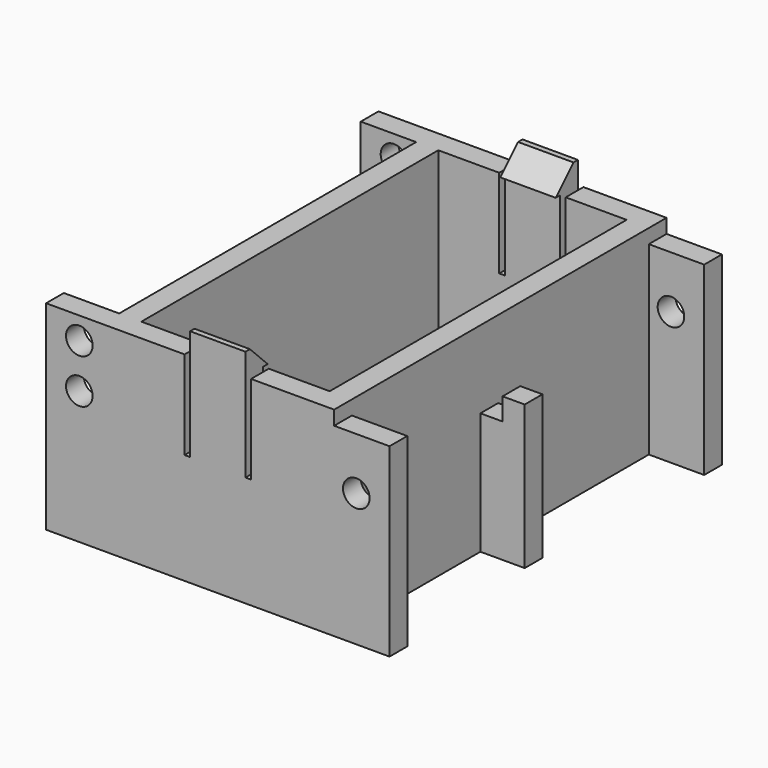
from build123d import *

# Parameters (mm, degrees)
F1_DEPTH  = 2
F2_DEPTH  = 18
F3_DEPTH  = 3
F4_W      = 2
F4_H      = 5
F4_H_2    = 13
F5_DEPTH  = 5
F6_W      = 2
F6_H      = 16.7173967883
F7_DEPTH  = 5
F8_R      = 1.2
F9_DEPTH  = 40
F12_DEPTH = 1
F13_W     = 5
F13_H     = 2
F13_H_2   = 0.5
F14_DEPTH = 2
F15_SIZE  = 1.99999
F13_W_2   = 0.5
F16_DEPTH = 8


# Not quite as in the source:
# - a fillet or chamfer is up to 0.001 mm smaller than in the source, because OpenCascade refuses the exact size


with BuildPart() as f1:
    # F0 (on Top) → F1 (new body)
    with BuildSketch(Plane.XY):
        Polygon((-5.1606558692, 9.7513413054), (-11.6606558692, 9.7513413054), (-11.6606558692, -27.7486586946), (-5.1606558692, -27.7486586946), (2.8393441308, -27.7486586946), (9.3393441308, -27.7486586946), (9.3393441308, 9.7513413054), (2.8393441308, 9.7513413054), align=None)
        Polygon((-9.6606558692, -1.2486586946), (-9.6606558692, 7.7513413054), (7.3393441308, 7.7513413054), (7.3393441308, -1.2486586946), (7.3393441308, -16.7486586946), (7.3393441308, -25.7486586946), (-9.6606558692, -25.7486586946), (-9.6606558692, -16.7486586946), align=None, mode=Mode.SUBTRACT)
        with BuildLine():
            Line((3.3125979801, -16.7486586946), (-5.6339097184, -16.7486586946))
            ThreePointArc((-5.6339097184, -16.7486586946), (-2.8409986659, -25.1856853401), (4.3393441308, -19.9486586946))
            ThreePointArc((4.3393441308, -19.9486586946), (4.0763707763, -18.2683158979), (3.3125979801, -16.7486586946))
        make_face()
        with BuildLine():
            ThreePointArc((4.3393441308, 1.9513413054), (-2.8409986659, 7.1883679509), (-5.6339097184, -1.2486586946))
            Line((-5.6339097184, -1.2486586946), (3.3125979801, -1.2486586946))
            ThreePointArc((3.3125979801, -1.2486586946), (4.0763707763, 0.2709985087), (4.3393441308, 1.9513413054))
        make_face()
        with BuildLine():
            Line((7.3393441308, 7.7513413054), (-9.6606558692, 7.7513413054))
            Line((-9.6606558692, 7.7513413054), (-9.6606558692, -1.2486586946))
            Line((-9.6606558692, -1.2486586946), (-5.6339097184, -1.2486586946))
            ThreePointArc((-5.6339097184, -1.2486586946), (-2.8409986659, 7.1883679509), (4.3393441308, 1.9513413054))
            ThreePointArc((4.3393441308, 1.9513413054), (4.0763707763, 0.2709985087), (3.3125979801, -1.2486586946))
            Line((3.3125979801, -1.2486586946), (7.3393441308, -1.2486586946))
            Line((7.3393441308, -1.2486586946), (7.3393441308, 7.7513413054))
        make_face()
        with BuildLine():
            Line((-5.6339097184, -16.7486586946), (-9.6606558692, -16.7486586946))
            Line((-9.6606558692, -16.7486586946), (-9.6606558692, -25.7486586946))
            Line((-9.6606558692, -25.7486586946), (7.3393441308, -25.7486586946))
            Line((7.3393441308, -25.7486586946), (7.3393441308, -16.7486586946))
            Line((7.3393441308, -16.7486586946), (3.3125979801, -16.7486586946))
            ThreePointArc((3.3125979801, -16.7486586946), (4.0763707763, -18.2683158979), (4.3393441308, -19.9486586946))
            ThreePointArc((4.3393441308, -19.9486586946), (-2.8409986659, -25.1856853401), (-5.6339097184, -16.7486586946))
        make_face()
        with BuildLine():
            Line((7.3393441308, -16.7486586946), (7.3393441308, -1.2486586946))
            Line((7.3393441308, -1.2486586946), (3.3125979801, -1.2486586946))
            ThreePointArc((3.3125979801, -1.2486586946), (2.6358545698, -2.028169781), (1.8253711817, -2.667494311))
            ThreePointArc((1.8253711817, -2.667494311), (4.751289215, -5.2504717566), (5.8393441308, -8.9986586946))
            ThreePointArc((5.8393441308, -8.9986586946), (4.751289215, -12.7468456326), (1.8253711817, -15.3298230782))
            ThreePointArc((1.8253711817, -15.3298230782), (2.6358545698, -15.9691476082), (3.3125979801, -16.7486586946))
            Line((3.3125979801, -16.7486586946), (7.3393441308, -16.7486586946))
        make_face()
        with BuildLine():
            Line((-5.6339097184, -1.2486586946), (-9.6606558692, -1.2486586946))
            Line((-9.6606558692, -1.2486586946), (-9.6606558692, -16.7486586946))
            Line((-9.6606558692, -16.7486586946), (-5.6339097184, -16.7486586946))
            ThreePointArc((-5.6339097184, -16.7486586946), (-4.9571663082, -15.9691476082), (-4.14668292, -15.3298230782))
            ThreePointArc((-4.14668292, -15.3298230782), (-8.1606558692, -8.9986586946), (-4.14668292, -2.667494311))
            ThreePointArc((-4.14668292, -2.667494311), (-4.9571663082, -2.028169781), (-5.6339097184, -1.2486586946))
        make_face()
        with BuildLine():
            Line((3.3125979801, -1.2486586946), (-5.6339097184, -1.2486586946))
            ThreePointArc((-5.6339097184, -1.2486586946), (-4.9571663082, -2.028169781), (-4.14668292, -2.667494311))
            ThreePointArc((-4.14668292, -2.667494311), (-1.1606558692, -1.9986586946), (1.8253711817, -2.667494311))
            ThreePointArc((1.8253711817, -2.667494311), (2.6358545698, -2.028169781), (3.3125979801, -1.2486586946))
        make_face()
        with BuildLine():
            ThreePointArc((-4.14668292, -15.3298230782), (-4.9571663082, -15.9691476082), (-5.6339097184, -16.7486586946))
            Line((-5.6339097184, -16.7486586946), (3.3125979801, -16.7486586946))
            ThreePointArc((3.3125979801, -16.7486586946), (2.6358545698, -15.9691476082), (1.8253711817, -15.3298230782))
            ThreePointArc((1.8253711817, -15.3298230782), (-1.1606558692, -15.9986586946), (-4.14668292, -15.3298230782))
        make_face()
    extrude(amount=F1_DEPTH)

    # F0 (on Top) → F2 (join)
    with BuildSketch(Plane.XY):
        Polygon((-5.1606558692, 9.7513413054), (-11.6606558692, 9.7513413054), (-11.6606558692, -27.7486586946), (-5.1606558692, -27.7486586946), (2.8393441308, -27.7486586946), (9.3393441308, -27.7486586946), (9.3393441308, 9.7513413054), (2.8393441308, 9.7513413054), align=None)
        Polygon((-9.6606558692, -1.2486586946), (-9.6606558692, 7.7513413054), (7.3393441308, 7.7513413054), (7.3393441308, -1.2486586946), (7.3393441308, -16.7486586946), (7.3393441308, -25.7486586946), (-9.6606558692, -25.7486586946), (-9.6606558692, -16.7486586946), align=None, mode=Mode.SUBTRACT)
    extrude(amount=F2_DEPTH)

    # F0 (on Top) → F3 (join)
    with BuildSketch(Plane.XY):
        with BuildLine():
            ThreePointArc((-3.604859431, -2.9757134891), (-3.8801412786, -2.8292861752), (-4.14668292, -2.667494311))
            ThreePointArc((-4.14668292, -2.667494311), (-8.1606558692, -8.9986586946), (-4.14668292, -15.3298230782))
            ThreePointArc((-4.14668292, -15.3298230782), (-3.8801412786, -15.1680312141), (-3.604859431, -15.0216039001))
            ThreePointArc((-3.604859431, -15.0216039001), (-7.6606558692, -8.9986586946), (-3.604859431, -2.9757134891))
        make_face()
        with BuildLine():
            ThreePointArc((1.8253711817, -2.667494311), (-1.1606558692, -1.9986586946), (-4.14668292, -2.667494311))
            ThreePointArc((-4.14668292, -2.667494311), (-3.8801412786, -2.8292861752), (-3.604859431, -2.9757134891))
            ThreePointArc((-3.604859431, -2.9757134891), (-1.1606558692, -2.4986586946), (1.2835476927, -2.9757134891))
            ThreePointArc((1.2835476927, -2.9757134891), (1.5588295403, -2.8292861752), (1.8253711817, -2.667494311))
        make_face()
        with BuildLine():
            ThreePointArc((5.8393441308, -8.9986586946), (4.751289215, -5.2504717566), (1.8253711817, -2.667494311))
            ThreePointArc((1.8253711817, -2.667494311), (1.5588295403, -2.8292861752), (1.2835476927, -2.9757134891))
            ThreePointArc((1.2835476927, -2.9757134891), (4.2308802362, -5.3680473929), (5.3393441308, -8.9986586946))
            ThreePointArc((5.3393441308, -8.9986586946), (4.2308802362, -12.6292699963), (1.2835476927, -15.0216039001))
            ThreePointArc((1.2835476927, -15.0216039001), (1.5588295403, -15.1680312141), (1.8253711817, -15.3298230782))
            ThreePointArc((1.8253711817, -15.3298230782), (4.751289215, -12.7468456326), (5.8393441308, -8.9986586946))
        make_face()
        with BuildLine():
            ThreePointArc((-3.604859431, -15.0216039001), (-3.8801412786, -15.1680312141), (-4.14668292, -15.3298230782))
            ThreePointArc((-4.14668292, -15.3298230782), (-1.1606558692, -15.9986586946), (1.8253711817, -15.3298230782))
            ThreePointArc((1.8253711817, -15.3298230782), (1.5588295403, -15.1680312141), (1.2835476927, -15.0216039001))
            ThreePointArc((1.2835476927, -15.0216039001), (-1.1606558692, -15.4986586946), (-3.604859431, -15.0216039001))
        make_face()
    extrude(amount=F3_DEPTH)

    # F4 (on face) → F5 (join)
    with BuildSketch(Plane(origin=(-11.6606558692, 0, 0), x_dir=(0, -1, 0), z_dir=(-1, 0, 0))):
        with Locations((-8.7513413054, 2.5)):
            Rectangle(F4_W, F4_H)
        with Locations((-8.7513413054, 11.5)):
            Rectangle(F4_W, F4_H_2)
        with Locations((26.7486586946, 2.5)):
            Rectangle(F4_W, F4_H)
        with Locations((26.7486586946, 11.5)):
            Rectangle(F4_W, F4_H_2)
    extrude(amount=F5_DEPTH)

    # F6 (on face) → F7 (join)
    with BuildSketch(Plane.YZ.offset(9.3393441308)):
        with Locations((-26.7486586946, 8.3586983941)):
            Rectangle(F6_W, F6_H)
        with Locations((8.7513413054, 8.3586983941)):
            Rectangle(F6_W, F6_H)
    extrude(amount=F7_DEPTH)

    # F8 (on face) → F9 (cut)
    with BuildSketch(Plane.XZ.offset(27.7486586946)):
        with Locations((-13.6606558692, 12)):
            Circle(F8_R)
        with Locations((11.3393441308, 12)):
            Circle(F8_R)
        with Locations((-13.6606558692, 16)):
            Circle(F8_R)
    extrude(amount=-F9_DEPTH, mode=Mode.SUBTRACT)

    # F11 (on offset) → F12 (join, symmetric)
    with BuildSketch(Plane(origin=(0, -10.2486586946, 0), x_dir=(-1, 0, 0), z_dir=(0, 1, 0))):
        Polygon((-13.3393441308, 13), (-13.3393441308, 0), (-9.3393441308, 0), (-9.3393441308, 11), (-11.3393441308, 11), (-11.3393441308, 13), align=None)
    extrude(amount=F12_DEPTH, both=True)

    # F13 (on face) → F14 (join)
    with BuildSketch(Plane.XY.offset(18)):
        with Locations((-1.1606558692, -26.7486586946)):
            Rectangle(F13_W, F13_H)
        with Locations((-1.1606558692, -25.4986586946)):
            Rectangle(F13_W, F13_H_2)
        with Locations((-1.1606558692, 8.7513413054)):
            Rectangle(F13_W, F13_H)
        with Locations((-1.1606558692, 7.5013413054)):
            Rectangle(F13_W, F13_H_2)
    extrude(amount=F14_DEPTH)

    # F15 (size 2 in the source; OpenCascade refuses exactly that, so slightly less here)
    f15_edges = [f1.edges().sort_by_distance(p)[0] for p in [
        (-1.160656, -25.248659, 20),
        (-1.160656, 7.251341, 20),
    ]]
    chamfer(f15_edges, length=F15_SIZE)

    # F13 (on face) → F16 (cut)
    with BuildSketch(Plane.XY.offset(18)):
        with Locations((-3.9106558692, -26.7486586946)):
            Rectangle(F13_W_2, F13_H)
        with Locations((1.5893441308, -26.7486586946)):
            Rectangle(F13_W_2, F13_H)
        with Locations((1.5893441308, 8.7513413054)):
            Rectangle(F13_W_2, F13_H)
        with Locations((-3.9106558692, 8.7513413054)):
            Rectangle(F13_W_2, F13_H)
    extrude(amount=-F16_DEPTH, mode=Mode.SUBTRACT)


solid = f1.part
